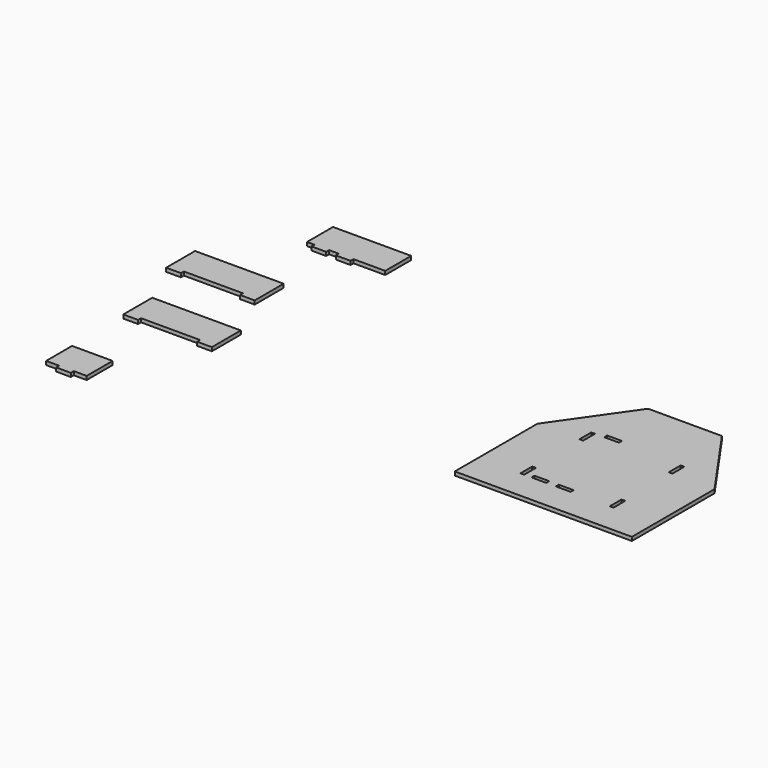
from build123d import *

# Parameters (mm, degrees)
F2_DEPTH = 3.175
F0_W     = 3.175
F0_H     = 12.7
F3_DEPTH = 3.175


# Not quite as in the source:
# - a feature names something its author has since deleted; it is built from what else it names


with BuildPart() as f2:
    # F1 (on Top) → F2 (new body)
    with BuildSketch(Plane.XY):
        Polygon((-273.056358099, 116.3102710271), (-340.366358099, 116.3102710271), (-340.366358099, 88.3702710271), (-334.016358099, 88.3702710271), (-334.016358099, 85.1952710271), (-321.316358099, 85.1952710271), (-321.316358099, 88.3702710271), (-313.061358099, 88.3702710271), (-313.061358099, 85.1952710271), (-300.361358099, 85.1952710271), (-300.361358099, 88.3702710271), (-273.056358099, 88.3702710271), align=None)
    extrude(amount=F2_DEPTH)


with BuildPart() as f2b:
    # F1 (on Top) → F2, piece 2 (new body)
    with BuildSketch(Plane.XY):
        Polygon((-314.6848678589, 31.115), (-390.8848678589, 31.115), (-390.8848678589, 3.175), (-390.8848678589, 0), (-378.1848678589, 0), (-378.1848678589, 3.175), (-327.3848678589, 3.175), (-327.3848678589, 0), (-314.6848678589, 0), (-314.6848678589, 3.175), align=None)
    extrude(amount=F2_DEPTH)


with BuildPart() as f2c:
    # F1 (on Top) → F2, piece 3 (new body)
    with BuildSketch(Plane.XY):
        Polygon((-294.6711480618, -39.9599104619), (-370.8711480618, -39.9599104619), (-370.8711480618, -67.8999104619), (-370.8711480618, -71.0749104619), (-358.1711480618, -71.0749104619), (-358.1711480618, -67.8999104619), (-307.3711480618, -67.8999104619), (-307.3711480618, -71.0749104619), (-294.6711480618, -71.0749104619), (-294.6711480618, -67.8999104619), align=None)
    extrude(amount=F2_DEPTH)


with BuildPart() as f2d:
    # F1 (on Top) → F2, piece 4 (new body)
    with BuildSketch(Plane.XY):
        Polygon((-334.2218278885, -128.3455094671), (-369.1468278885, -128.3455094671), (-369.1468278885, -156.2855094671), (-358.0343278885, -156.2855094671), (-358.0343278885, -159.4605094671), (-345.3343278885, -159.4605094671), (-345.3343278885, -156.2855094671), (-334.2218278885, -156.2855094671), align=None)
    extrude(amount=F2_DEPTH)


with BuildPart() as f3:
    # F0 (on Top) → F3 (new body)
    with BuildSketch(Plane.XY):
        Polygon((-54.2813502252, -26.5063998628), (-54.2813502252, -110.3263998628), (-41.5813502252, -110.3263998628), (-18.0863502252, -110.3263998628), (0, -110.3263998628), (21.9186497748, -110.3263998628), (53.6686497748, -110.3263998628), (85.4186497748, -110.3263998628), (98.1186497748, -110.3263998628), (98.1186497748, -98.0041697621), (98.1186497748, -34.1263998628), (98.1186497748, -26.5063998628), (98.1186497748, -21.4263998628), (53.6686497748, 42.0736001372), (-9.8313502252, 42.0736001372), (-54.2813502252, -21.4263998628), align=None)
        with Locations((-16.4988502252, -78.5763998628)):
            Rectangle(F0_W, F0_H, mode=Mode.SUBTRACT)
        Polygon((4.1386497748, -84.9263998628), (-2.2113502252, -84.9263998628), (-8.5613502252, -84.9263998628), (-8.5613502252, -81.7513998628), (4.1386497748, -81.7513998628), align=None, mode=Mode.SUBTRACT)
        Polygon((25.0936497748, -84.9263998628), (18.7436497748, -84.9263998628), (12.3936497748, -84.9263998628), (12.3936497748, -81.7513998628), (25.0936497748, -81.7513998628), align=None, mode=Mode.SUBTRACT)
        with Locations((60.3361497748, -78.5763998628)):
            Rectangle(F0_W, F0_H, mode=Mode.SUBTRACT)
        with Locations((-16.4988502252, -15.0763998628)):
            Rectangle(F0_W, F0_H, mode=Mode.SUBTRACT)
        Polygon((5.7261497748, -8.7263998628), (-0.6238502252, -8.7263998628), (-6.9738502252, -8.7263998628), (-6.9738502252, -5.5513998628), (5.7261497748, -5.5513998628), align=None, mode=Mode.SUBTRACT)
        with Locations((60.3361497748, -15.0763998628)):
            Rectangle(F0_W, F0_H, mode=Mode.SUBTRACT)
    extrude(amount=F3_DEPTH)


solid = Compound([f2.part, f2b.part, f2c.part, f2d.part, f3.part])
